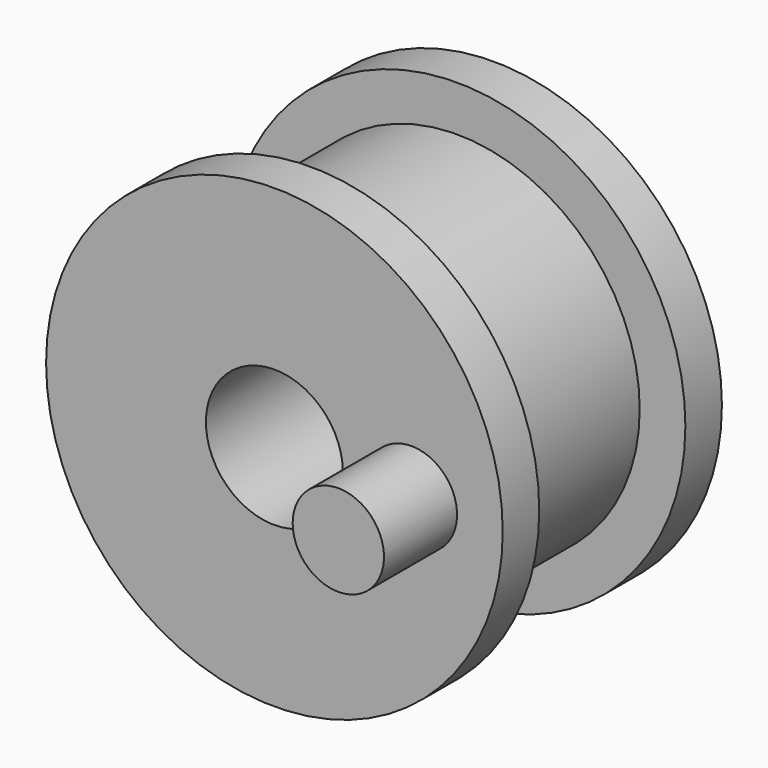
from build123d import *

# Parameters (mm, degrees)
F0_R     = 12.7
F1_DEPTH = 12.7
F2_R     = 15.875
F2_R_2   = 12.7
F3_DEPTH = 3.175
F4_R     = 15.875
F4_R_2   = 12.7
F5_DEPTH = 3.175
F7_DEPTH = 6.35
F8_R     = 4.7625
F9_DEPTH = 50.8


with BuildPart() as f1:
    # F0 (on Front) → F1 (new body)
    with BuildSketch(Plane.XZ):
        Circle(F0_R)
    extrude(amount=F1_DEPTH)

    # F2 (on face) → F3 (join)
    with BuildSketch(Plane.XZ.offset(12.7)):
        Circle(F2_R)
        Circle(F2_R_2, mode=Mode.SUBTRACT)
        Circle(F2_R_2)
    extrude(amount=F3_DEPTH)

    # F4 (on face) → F5 (join)
    with BuildSketch(Plane(origin=(0, 0, 0), x_dir=(-1, 0, 0), z_dir=(0, 1, 0))):
        Circle(F4_R)
        Circle(F4_R_2, mode=Mode.SUBTRACT)
        Circle(F4_R_2)
    extrude(amount=F5_DEPTH)

    # F6 (on face) → F7 (join)
    with BuildSketch(Plane.XZ.offset(15.875)):
        with BuildLine():
            ThreePointArc((12.7, 0), (9.525, 3.175), (6.35, 0))
            ThreePointArc((6.35, 0), (9.525, -3.175), (12.7, 0))
        make_face()
    extrude(amount=F7_DEPTH)

    # F8 (on face) → F9 (cut)
    with BuildSketch(Plane.XZ.offset(15.875)):
        Circle(F8_R)
    extrude(amount=-F9_DEPTH, mode=Mode.SUBTRACT)


solid = f1.part
